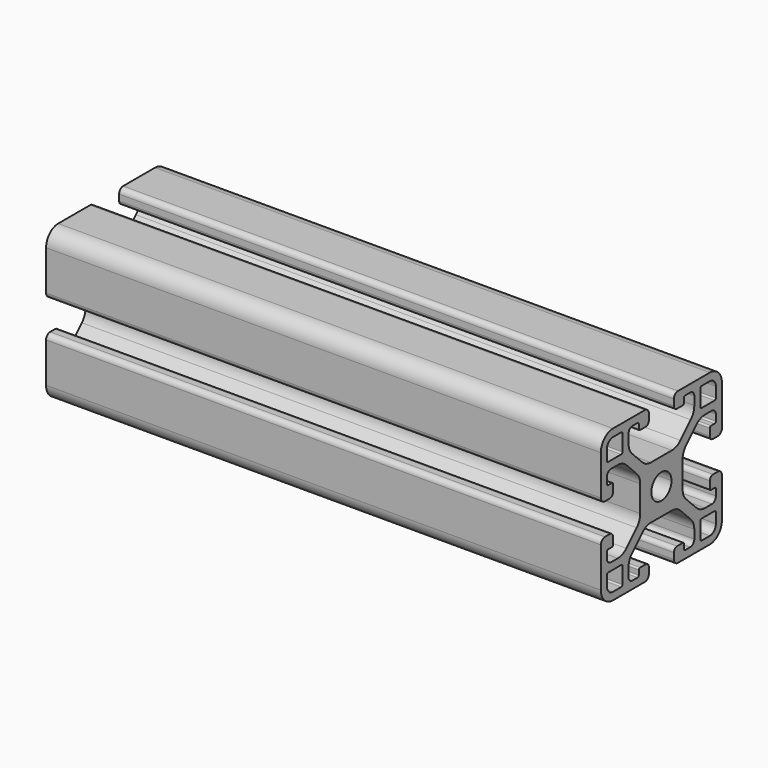
from build123d import *

# Parameters (mm, degrees)
F1_DEPTH = 55


# Not quite as in the source:
# - ends of sketch curves that miss each other by under 0.0002 mm in the source are joined


with BuildPart() as f1:
    # F0 (on Right) → F1 (new body, symmetric)
    with BuildSketch(Plane.YZ):
        with BuildLine():
            ThreePointArc((10.806854, -8.15), (9.6588037029, -7.9216385975), (8.6855336564, -7.2713203436))
            Line((8.6855336564, -7.2713203436), (6.128679, -4.714466))
            ThreePointArc((6.128679, -4.714466), (5.4783614025, -3.7411962971), (5.25, -2.593146))
            Line((5.25, -2.593146), (5.25, 0))
            Line((5.25, 0), (2.5, 0))
            ThreePointArc((2.5, 0), (1.767766953, -1.767766953), (0, -2.5))
            Line((0, -2.5), (0, -5.25))
            Line((0, -5.25), (2.593145, -5.25))
            ThreePointArc((2.593145, -5.25), (3.7411962971, -5.4783614025), (4.7144663436, -6.1286796564))
            Line((4.7144663436, -6.1286796564), (7.27132, -8.685534))
            ThreePointArc((7.27132, -8.685534), (7.9216385975, -9.6588037029), (8.15, -10.806854))
            Line((8.15, -10.806854), (8.15, -12.5))
            ThreePointArc((8.15, -12.5), (7.8571067812, -13.2071067812), (7.15, -13.5))
            Line((7.15, -13.5), (5.9, -13.5))
            ThreePointArc((5.9, -13.5), (5.6878679656, -13.4121320344), (5.6, -13.2))
            Line((5.6, -13.2), (5.6, -12.3))
            ThreePointArc((5.6, -12.3), (5.5121320344, -12.0878679656), (5.3, -12))
            Line((5.3, -12), (3.9, -12))
            ThreePointArc((3.9, -12), (3.3343145751, -12.2343145751), (3.1, -12.8))
            Line((3.1, -12.8), (3.1, -14))
            ThreePointArc((3.1, -14), (3.3928932188, -14.7071067812), (4.1, -15))
            Line((4.1, -15), (12, -15))
            ThreePointArc((12, -15), (14.1213203436, -14.1213203436), (15, -12))
            Line((15, -12), (15, -4.1))
            ThreePointArc((15, -4.1), (14.7071067812, -3.3928932188), (14, -3.1))
            Line((14, -3.1), (12.799999, -3.1))
            ThreePointArc((12.799999, -3.1), (12.2343145751, -3.3343145751), (12, -3.9))
            Line((12, -3.9), (12, -5.3))
            ThreePointArc((12, -5.3), (12.0878679656, -5.5121320344), (12.3, -5.6))
            Line((12.3, -5.6), (13.200001, -5.6))
            ThreePointArc((13.200001, -5.6), (13.4121320344, -5.6878679656), (13.5, -5.9))
            Line((13.5, -5.9), (13.5, -7.15))
            ThreePointArc((13.5, -7.15), (13.2071067812, -7.8571067812), (12.5, -8.15))
            Line((12.5, -8.15), (10.806854, -8.15))
        make_face()
        with BuildLine():
            Line((12, -13.5), (9.950001, -13.5))
            ThreePointArc((9.950001, -13.5), (9.7378679656, -13.4121320344), (9.65, -13.2))
            Line((9.65, -13.2), (9.65, -9.95))
            ThreePointArc((9.65, -9.95), (9.7378679656, -9.7378679656), (9.95, -9.65))
            Line((9.95, -9.65), (13.200001, -9.65))
            ThreePointArc((13.200001, -9.65), (13.4121320344, -9.7378679656), (13.5, -9.95))
            Line((13.5, -9.95), (13.5, -12))
            ThreePointArc((13.5, -12), (13.0606601718, -13.0606601718), (12, -13.5))
        make_face(mode=Mode.SUBTRACT)
        with BuildLine():
            Line((2.5, 0), (5.25, 0))
            Line((5.25, 0), (5.25, 2.593145))
            ThreePointArc((5.25, 2.593145), (5.4783614025, 3.7411962971), (6.1286796564, 4.7144663436))
            Line((6.1286796564, 4.7144663436), (8.685534, 7.27132))
            ThreePointArc((8.685534, 7.27132), (9.6588037029, 7.9216385975), (10.806854, 8.15))
            Line((10.806854, 8.15), (12.5, 8.15))
            ThreePointArc((12.5, 8.15), (13.2071067812, 7.8571067812), (13.5, 7.15))
            Line((13.5, 7.15), (13.5, 5.9))
            ThreePointArc((13.5, 5.9), (13.4121320344, 5.6878679656), (13.2, 5.6))
            Line((13.2, 5.6), (12.299999, 5.6))
            ThreePointArc((12.299999, 5.6), (12.0878679656, 5.5121320344), (12, 5.3))
            Line((12, 5.3), (12, 3.9))
            ThreePointArc((12, 3.9), (12.2343145751, 3.3343145751), (12.8, 3.1))
            Line((12.8, 3.1), (14, 3.1))
            ThreePointArc((14, 3.1), (14.7071067812, 3.3928932188), (15, 4.1))
            Line((15, 4.1), (15, 12))
            ThreePointArc((15, 12), (14.1213203436, 14.1213203436), (12, 15))
            Line((12, 15), (4.1, 15))
            ThreePointArc((4.1, 15), (3.3928932188, 14.7071067812), (3.1, 14))
            Line((3.1, 14), (3.1, 12.799999))
            ThreePointArc((3.1, 12.799999), (3.3343145751, 12.2343145751), (3.9, 12))
            Line((3.9, 12), (5.299999, 12))
            ThreePointArc((5.299999, 12), (5.5121320344, 12.0878679656), (5.6, 12.3))
            Line((5.6, 12.3), (5.6, 13.200001))
            ThreePointArc((5.6, 13.200001), (5.6878679656, 13.4121320344), (5.9, 13.5))
            Line((5.9, 13.5), (7.15, 13.5))
            ThreePointArc((7.15, 13.5), (7.8571067812, 13.2071067812), (8.15, 12.5))
            Line((8.15, 12.5), (8.15, 10.806854))
            ThreePointArc((8.15, 10.806854), (7.9216385975, 9.6588037029), (7.2713203436, 8.6855336564))
            Line((7.2713203436, 8.6855336564), (4.714466, 6.128679))
            ThreePointArc((4.714466, 6.128679), (3.7411962971, 5.4783614025), (2.593146, 5.25))
            Line((2.593146, 5.25), (0, 5.25))
            Line((0, 5.25), (0, 2.5))
            ThreePointArc((0, 2.5), (1.767766953, 1.767766953), (2.5, 0))
        make_face()
        with BuildLine():
            Line((13.200001, 9.65), (9.950001, 9.65))
            ThreePointArc((9.950001, 9.65), (9.7378679656, 9.7378679656), (9.65, 9.95))
            Line((9.65, 9.95), (9.65, 13.200001))
            ThreePointArc((9.65, 13.200001), (9.7378679656, 13.4121320344), (9.95, 13.5))
            Line((9.95, 13.5), (12, 13.5))
            ThreePointArc((12, 13.5), (13.0606601718, 13.0606601718), (13.5, 12))
            Line((13.5, 12), (13.5, 9.950001))
            ThreePointArc((13.5, 9.950001), (13.4121320344, 9.7378679656), (13.200001, 9.65))
        make_face(mode=Mode.SUBTRACT)
        with BuildLine():
            ThreePointArc((-2.5, 0), (-1.767766953, 1.767766953), (0, 2.5))
            Line((0, 2.5), (0, 5.25))
            Line((0, 5.25), (-2.593145, 5.25))
            ThreePointArc((-2.593145, 5.25), (-3.7411962971, 5.4783614025), (-4.7144663436, 6.1286796564))
            Line((-4.7144663436, 6.1286796564), (-7.27132, 8.685534))
            ThreePointArc((-7.27132, 8.685534), (-7.9216385975, 9.6588037029), (-8.15, 10.806854))
            Line((-8.15, 10.806854), (-8.15, 12.5))
            ThreePointArc((-8.15, 12.5), (-7.8571067812, 13.2071067812), (-7.15, 13.5))
            Line((-7.15, 13.5), (-5.9, 13.5))
            ThreePointArc((-5.9, 13.5), (-5.6878679656, 13.4121320344), (-5.6, 13.2))
            Line((-5.6, 13.2), (-5.6, 12.299999))
            ThreePointArc((-5.6, 12.299999), (-5.5121320344, 12.0878679656), (-5.3, 12))
            Line((-5.3, 12), (-3.9, 12))
            ThreePointArc((-3.9, 12), (-3.3343145751, 12.2343145751), (-3.1, 12.8))
            Line((-3.1, 12.8), (-3.1, 14))
            ThreePointArc((-3.1, 14), (-3.3928932188, 14.7071067812), (-4.1, 15))
            Line((-4.1, 15), (-12, 15))
            ThreePointArc((-12, 15), (-14.1213203436, 14.1213203436), (-15, 12))
            Line((-15, 12), (-15, 4.1))
            ThreePointArc((-15, 4.1), (-14.7071067812, 3.3928932188), (-14, 3.1))
            Line((-14, 3.1), (-12.8, 3.1))
            ThreePointArc((-12.8, 3.1), (-12.2343145751, 3.3343145751), (-12, 3.9))
            Line((-12, 3.9), (-12, 5.299999))
            ThreePointArc((-12, 5.299999), (-12.0878679656, 5.5121320344), (-12.3, 5.6))
            Line((-12.3, 5.6), (-13.2, 5.6))
            ThreePointArc((-13.2, 5.6), (-13.4121320344, 5.6878679656), (-13.5, 5.9))
            Line((-13.5, 5.9), (-13.5, 7.15))
            ThreePointArc((-13.5, 7.15), (-13.2071067812, 7.8571067812), (-12.5, 8.15))
            Line((-12.5, 8.15), (-10.806854, 8.15))
            ThreePointArc((-10.806854, 8.15), (-9.6588037029, 7.9216385975), (-8.6855336564, 7.2713203436))
            Line((-8.6855336564, 7.2713203436), (-6.128679, 4.714466))
            ThreePointArc((-6.128679, 4.714466), (-5.4783614025, 3.7411962971), (-5.25, 2.593146))
            Line((-5.25, 2.593146), (-5.25, 0))
            Line((-5.25, 0), (-2.5, 0))
        make_face()
        with BuildLine():
            Line((-9.95, 9.65), (-13.2, 9.65))
            ThreePointArc((-13.2, 9.65), (-13.4121320344, 9.7378679656), (-13.5, 9.95))
            Line((-13.5, 9.95), (-13.5, 12))
            ThreePointArc((-13.5, 12), (-13.0606601718, 13.0606601718), (-12, 13.5))
            Line((-12, 13.5), (-9.95, 13.5))
            ThreePointArc((-9.95, 13.5), (-9.7378679656, 13.4121320344), (-9.65, 13.2))
            Line((-9.65, 13.2), (-9.65, 9.950001))
            ThreePointArc((-9.65, 9.950001), (-9.7378679656, 9.7378679656), (-9.95, 9.65))
        make_face(mode=Mode.SUBTRACT)
        with BuildLine():
            Line((0, -5.25), (0, -2.5))
            ThreePointArc((0, -2.5), (-1.767766953, -1.767766953), (-2.5, 0))
            Line((-2.5, 0), (-5.25, 0))
            Line((-5.25, 0), (-5.25, -2.593145))
            ThreePointArc((-5.25, -2.593145), (-5.4783614025, -3.7411962971), (-6.1286796564, -4.7144663436))
            Line((-6.1286796564, -4.7144663436), (-8.685534, -7.27132))
            ThreePointArc((-8.685534, -7.27132), (-9.6588037029, -7.9216385975), (-10.806854, -8.15))
            Line((-10.806854, -8.15), (-12.5, -8.15))
            ThreePointArc((-12.5, -8.15), (-13.2071067812, -7.8571067812), (-13.5, -7.15))
            Line((-13.5, -7.15), (-13.5, -5.9))
            ThreePointArc((-13.5, -5.9), (-13.4121320344, -5.6878679656), (-13.2, -5.6))
            Line((-13.2, -5.6), (-12.3, -5.6))
            ThreePointArc((-12.3, -5.6), (-12.0878679656, -5.5121320344), (-12, -5.3))
            Line((-12, -5.3), (-12, -3.9))
            ThreePointArc((-12, -3.9), (-12.2343145751, -3.3343145751), (-12.8, -3.1))
            Line((-12.8, -3.1), (-14, -3.1))
            ThreePointArc((-14, -3.1), (-14.7071067812, -3.3928932188), (-15, -4.1))
            Line((-15, -4.1), (-15, -12))
            ThreePointArc((-15, -12), (-14.1213203436, -14.1213203436), (-12, -15))
            Line((-12, -15), (-4.1, -15))
            ThreePointArc((-4.1, -15), (-3.3928932188, -14.7071067812), (-3.1, -14))
            Line((-3.1, -14), (-3.1, -12.8))
            ThreePointArc((-3.1, -12.8), (-3.3343145751, -12.2343145751), (-3.9, -12))
            Line((-3.9, -12), (-5.3, -12))
            ThreePointArc((-5.3, -12), (-5.5121320344, -12.0878679656), (-5.6, -12.3))
            Line((-5.6, -12.3), (-5.6, -13.2))
            ThreePointArc((-5.6, -13.2), (-5.6878679656, -13.4121320344), (-5.9, -13.5))
            Line((-5.9, -13.5), (-7.15, -13.5))
            ThreePointArc((-7.15, -13.5), (-7.8571067812, -13.2071067812), (-8.15, -12.5))
            Line((-8.15, -12.5), (-8.15, -10.806854))
            ThreePointArc((-8.15, -10.806854), (-7.9216385975, -9.6588037029), (-7.2713203436, -8.6855336564))
            Line((-7.2713203436, -8.6855336564), (-4.714466, -6.128679))
            ThreePointArc((-4.714466, -6.128679), (-3.7411962971, -5.4783614025), (-2.593146, -5.25))
            Line((-2.593146, -5.25), (0, -5.25))
        make_face()
        with BuildLine():
            Line((-9.95, -13.5), (-12, -13.5))
            ThreePointArc((-12, -13.5), (-13.0606601718, -13.0606601718), (-13.5, -12))
            Line((-13.5, -12), (-13.5, -9.95))
            ThreePointArc((-13.5, -9.95), (-13.4121320344, -9.7378679656), (-13.2, -9.65))
            Line((-13.2, -9.65), (-9.95, -9.65))
            ThreePointArc((-9.95, -9.65), (-9.7378679656, -9.7378679656), (-9.65, -9.95))
            Line((-9.65, -9.95), (-9.65, -13.2))
            ThreePointArc((-9.65, -13.2), (-9.7378679656, -13.4121320344), (-9.95, -13.5))
        make_face(mode=Mode.SUBTRACT)
    extrude(amount=F1_DEPTH, both=True)


solid = f1.part
